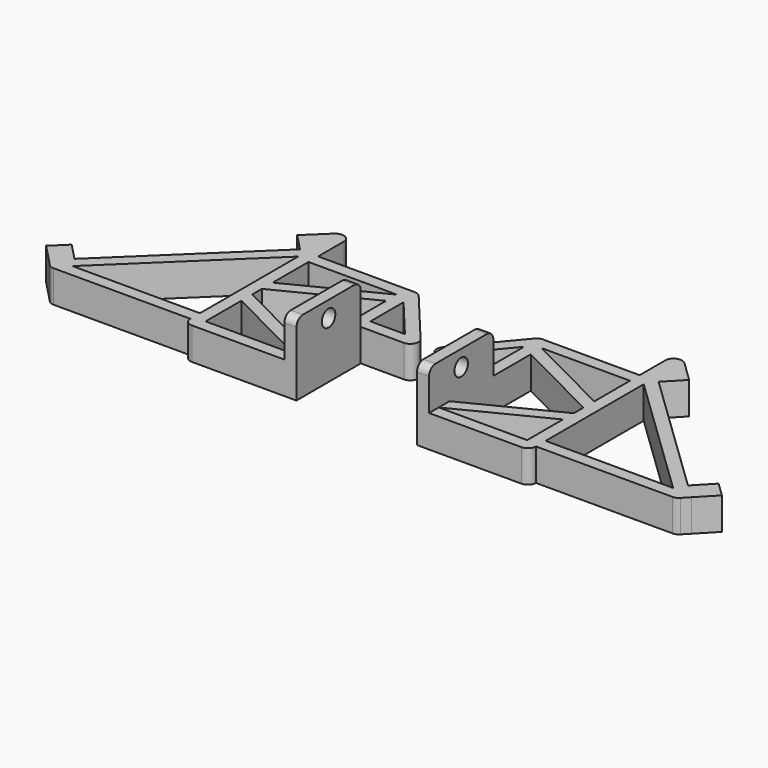
from build123d import *

# Parameters (mm, degrees)
F0_W     = 22
F0_H     = 3
F1_DEPTH = 8
F2_R     = 1.5
F3_DEPTH = 6.8
F4_W     = 3
F4_H     = 20
F5_DEPTH = 10
F6_R     = 1.99999
F7_R     = 2.1
F8_DEPTH = 15.7309281251


# Not quite as in the source:
# - a fillet or chamfer is up to 0.001 mm smaller than in the source, because OpenCascade refuses the exact size


with BuildPart() as f1:
    # F0 (on Top) → F1 (new body)
    with BuildSketch(Plane.XY):
        Polygon((-40, 28), (-43, 28), (-43, 19.6750785959), (-43, 15.5126178938), (-43, -15), (-43, -18), (-43, -20), (-40, -20), (-40, -17), (-40, -5.8625273576), (-40, -2.5), (-40, 0.5), (-40, 3.8625273576), (-40, 15), (-40, 18), align=None)
        Polygon((-43, 19.6750785959), (-43, 28), (-48.7658202006, 22.4542523124), (-44.6065094348, 18.129887162), align=None)
        Polygon((-43, 15.5126178938), (-43, 19.6750785959), (-44.6065094348, 18.129887162), (-76.3185205379, -12.37172512), (-79.9221581632, -15.8378174248), (-77.8425027804, -18), (-74.7234534518, -15), align=None)
        with Locations((-29, 16.5)):
            Rectangle(F0_W, F0_H)
        Polygon((-43, -18), (-43, -15), (-74.7234534518, -15), (-77.8425027804, -18), align=None)
        Polygon((-79.9221581632, -15.8378174248), (-76.3185205379, -12.37172512), (-80.4778313036, -8.0473599696), (-84.081468929, -11.5134522744), align=None)
        Polygon((-15, 18), (-18, 18), (-18, 15), (-18, 11.6374726424), (-18, 0.5), (-18, -2.5), (-18, -13.6374726424), (-18, -17), (-18, -20), (-15, -20), (-15, 0), (-15, 3), (-15, 13.3138501945), align=None)
        Polygon((0, 0), (-15, 18), (-15, 13.3138501945), (-6.405124838, 3), (-15, 3), (-15, 0), align=None)
        with Locations((-29, -18.5)):
            Rectangle(F0_W, F0_H)
        Polygon((-18, -13.6374726424), (-40, -2.5), (-40, -5.8625273576), (-18, -17), align=None)
        Polygon((-18, 15), (-40, 3.8625273576), (-40, 0.5), (-18, 11.6374726424), align=None)
    extrude(amount=F1_DEPTH)

    # F2 (on face) → F3 (cut)
    with BuildSketch(Plane(origin=(-34.6531344076, 36.0282785359, 0), x_dir=(-0.7207275251, -0.693218461, 0), z_dir=(-0.693218461, 0.7207275251, 0))):
        with Locations((66.0811666713, 4)):
            Circle(F2_R)
        with Locations((16.5811666713, 4)):
            Circle(F2_R)
    extrude(amount=-F3_DEPTH, mode=Mode.SUBTRACT)

    # F4 (on face) → F5 (join)
    with BuildSketch(Plane.XY.offset(8)):
        with Locations((-16.5, -10)):
            Rectangle(F4_W, F4_H)
    extrude(amount=F5_DEPTH)

    # F6 (radius 2 in the source; OpenCascade refuses exactly that, so slightly less here)
    f6_edges = [f1.edges().sort_by_distance(p)[0] for p in [
        (0, 0, 4),
        (-43, -20, 4),
        (-40, 28, 4),
        (-43, 28, 4),
        (-77.842503, -18, 4),
        (-15, 18, 4),
        (-16.5, 0, 18),
        (-16.5, -20, 18),
    ]]
    fillet(f6_edges, radius=F6_R)

    # F7 (on face) → F8 (cut, through all)
    with BuildSketch(Plane(origin=(-18, 0, 0), x_dir=(0, -1, 0), z_dir=(-1, 0, 0))):
        with Locations((10, 14)):
            Circle(F7_R)
    extrude(amount=-F8_DEPTH, mode=Mode.SUBTRACT)


with BuildPart() as f9_1:
    # F9: instance of F1
    add(f1.part.mirror(Plane.YZ))


solid = Compound([f1.part, f9_1.part])
